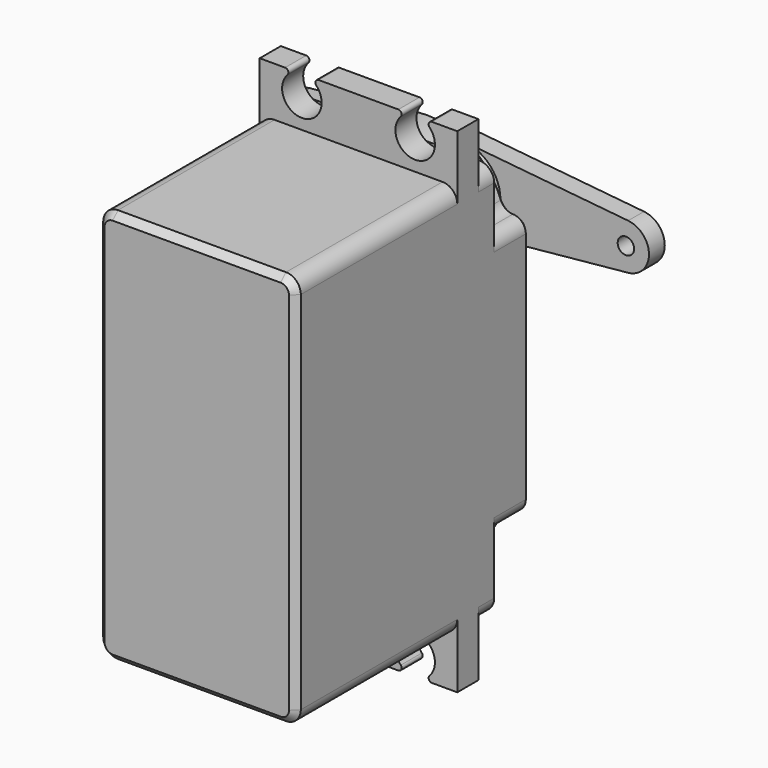
from build123d import *

# Parameters (mm, degrees)
F0_R      = 1.25
F1_DEPTH  = 3
F3_DEPTH  = 4
F4_R      = 3.475
F5_DEPTH  = 0.6
F6_R      = 1.5
F7_DEPTH  = 25
F8_R      = 3.7
F9_DEPTH  = 5
F10_R     = 3.975
F11_DEPTH = 6
F12_R     = 7.475
F13_DEPTH = 0.5
F15_DEPTH = 7
F16_R     = 2
F17_R     = 2
F18_W     = 30
F18_H     = 60
F19_DEPTH = 37.7
F21_W     = 30
F21_H     = 75
F22_DEPTH = 4
F23_R     = 2.25
F24_R     = 2.25
F25_SIZE  = 1
F26_R     = 3
F27_DEPTH = 25
F28_R     = 0.5
F29_SIZE  = 1


with BuildPart() as f1:
    # F0 (on Front) → F1 (new body)
    with BuildSketch(Plane.XZ):
        with BuildLine():
            Line((-25.343, -3.4831524514), (-0.5831, -5.9213591675))
            ThreePointArc((-0.5831, -5.9213591675), (0, -5.95), (0.5831, -5.9213591675))
            Line((0.5831, -5.9213591675), (25.343, -3.4831524514))
            ThreePointArc((25.343, -3.4831524514), (28.5, 0), (25.343, 3.4831524514))
            Line((25.343, 3.4831524514), (0.5831, 5.9213591675))
            ThreePointArc((0.5831, 5.9213591675), (0, 5.95), (-0.5831, 5.9213591675))
            Line((-0.5831, 5.9213591675), (-25.343, 3.4831524514))
            ThreePointArc((-25.343, 3.4831524514), (-28.5, 0), (-25.343, -3.4831524514))
        make_face()
        with Locations((-25, 0)):
            Circle(F0_R, mode=Mode.SUBTRACT)
        with Locations((25, 0)):
            Circle(F0_R, mode=Mode.SUBTRACT)
    extrude(amount=F1_DEPTH)

    # F2 (on face) → F3 (join)
    with BuildSketch(Plane.XZ.offset(3)):
        with BuildLine():
            ThreePointArc((0.5831, -5.9213591675), (4.4086247856, -3.9958137469), (5.95, 0))
            ThreePointArc((5.95, 0), (4.4086247856, 3.9958137469), (0.5831, 5.9213591675))
            ThreePointArc((0.5831, 5.9213591675), (0, 5.95), (-0.5831, 5.9213591675))
            ThreePointArc((-0.5831, 5.9213591675), (-5.95, 0), (-0.5831, -5.9213591675))
            ThreePointArc((-0.5831, -5.9213591675), (0, -5.95), (0.5831, -5.9213591675))
        make_face()
    extrude(amount=F3_DEPTH)

    # F4 (on face) → F5 (cut)
    with BuildSketch(Plane(origin=(0, 0, 0), x_dir=(-1, 0, 0), z_dir=(0, 1, 0))):
        Circle(F4_R)
    extrude(amount=-F5_DEPTH, mode=Mode.SUBTRACT)

    # F6 (on face) → F7 (cut)
    with BuildSketch(Plane(origin=(0, -0.6, 0), x_dir=(-1, 0, 0), z_dir=(0, 1, 0))):
        Circle(F6_R)
    extrude(amount=-F7_DEPTH, mode=Mode.SUBTRACT)

    # F8 (on face) → F9 (cut)
    with BuildSketch(Plane.XZ.offset(7)):
        Circle(F8_R)
    extrude(amount=-F9_DEPTH, mode=Mode.SUBTRACT)


with BuildPart() as f11:
    # F10 (on face) → F11 (new body)
    with BuildSketch(Plane.XZ.offset(2)):
        Circle(F10_R)
    extrude(amount=F11_DEPTH)

    # F12 (on face) → F13 (join)
    with BuildSketch(Plane.XZ.offset(8)):
        Circle(F12_R)
    extrude(amount=F13_DEPTH)

    # F14 (on face) → F15 (join)
    with BuildSketch(Plane.XZ.offset(8.5)):
        with BuildLine():
            Line((-11.6189500386, 3), (-15, 3))
            Line((-15, 3), (-15, -36.5))
            Line((-15, -36.5), (-11.6189500386, -36.5))
            ThreePointArc((-11.6189500386, -36.5), (0, -45.5), (11.6189500386, -36.5))
            Line((11.6189500386, -36.5), (15, -36.5))
            Line((15, -36.5), (15, 3))
            Line((15, 3), (11.6189500386, 3))
            ThreePointArc((11.6189500386, 3), (0, 12), (-11.6189500386, 3))
        make_face()
    extrude(amount=F15_DEPTH)

    # F16
    f16_edges = [f11.edges().sort_by_distance(p)[0] for p in [
        (-11.61895, -12, 3),
        (11.61895, -12, 3),
        (11.61895, -12, -36.5),
        (-11.61895, -12, -36.5),
    ]]
    fillet(f16_edges, radius=F16_R)

    # F17
    f17_edges = [f11.edges().sort_by_distance(p)[0] for p in [
        (15, -12, 3),
        (-15, -12, 3),
        (15, -12, -36.5),
        (-15, -12, -36.5),
    ]]
    fillet(f17_edges, radius=F17_R)

    # F18 (on face) → F19 (join)
    with BuildSketch(Plane.XZ.offset(15.5)):
        with Locations((0, -17.5)):
            Rectangle(F18_W, F18_H)
    extrude(amount=F19_DEPTH)

    # F21 (on offset) → F22 (join)
    with BuildSketch(Plane(origin=(0, -18.5, 0), x_dir=(-1, 0, 0), z_dir=(0, 1, 0))):
        with Locations((0, -17.5)):
            Rectangle(F21_W, F21_H)
    extrude(amount=-F22_DEPTH)

    # F23
    f23_edges = [f11.edges().sort_by_distance(p)[0] for p in [
        (15, -17, 12.5),
        (-15, -17, 12.5),
        (15, -17, -47.5),
        (-15, -17, -47.5),
    ]]
    fillet(f23_edges, radius=F23_R)

    # F24
    f24_edges = [f11.edges().sort_by_distance(p)[0] for p in [
        (15, -37.85, 12.5),
        (15, -37.85, -47.5),
        (-15, -37.85, -47.5),
        (-15, -37.85, 12.5),
    ]]
    fillet(f24_edges, radius=F24_R)

    # F25
    f25_edges = [f11.edges().sort_by_distance(p)[0] for p in [
        (0, -53.2, -47.5),
        (-14.34099, -53.2, -46.84099),
        (14.34099, -53.2, -46.84099),
        (-15, -53.2, -17.5),
        (15, -53.2, -17.5),
        (-14.34099, -53.2, 11.84099),
        (14.34099, -53.2, 11.84099),
        (0, -53.2, 12.5),
    ]]
    chamfer(f25_edges, length=F25_SIZE)

    # F26 (on face) → F27 (cut)
    with BuildSketch(Plane(origin=(0, -18.5, 0), x_dir=(-1, 0, 0), z_dir=(0, 1, 0))):
        with Locations((-8.6, -52.1)):
            Circle(F26_R)
        with Locations((-8.6, 17.1)):
            Circle(F26_R)
        with Locations((8.6, -52.1)):
            Circle(F26_R)
        with Locations((8.6, 17.1)):
            Circle(F26_R)
    extrude(amount=-F27_DEPTH, mode=Mode.SUBTRACT)

    # F28
    f28_edges = [f11.edges().sort_by_distance(p)[0] for p in [
        (9.368115, -20.5, -55),
        (7.831885, -20.5, -55),
        (-7.831885, -20.5, -55),
        (-9.368115, -20.5, -55),
        (9.368115, -20.5, 20),
        (7.831885, -20.5, 20),
        (-7.831885, -20.5, 20),
        (-9.368115, -20.5, 20),
    ]]
    fillet(f28_edges, radius=F28_R)

    # F29
    f29_edges = [f11.edges().sort_by_distance(p)[0] for p in [
        (-15, -8.5, -16.75),
    ]]
    chamfer(f29_edges, length=F29_SIZE)


solid = Compound([f1.part, f11.part])
